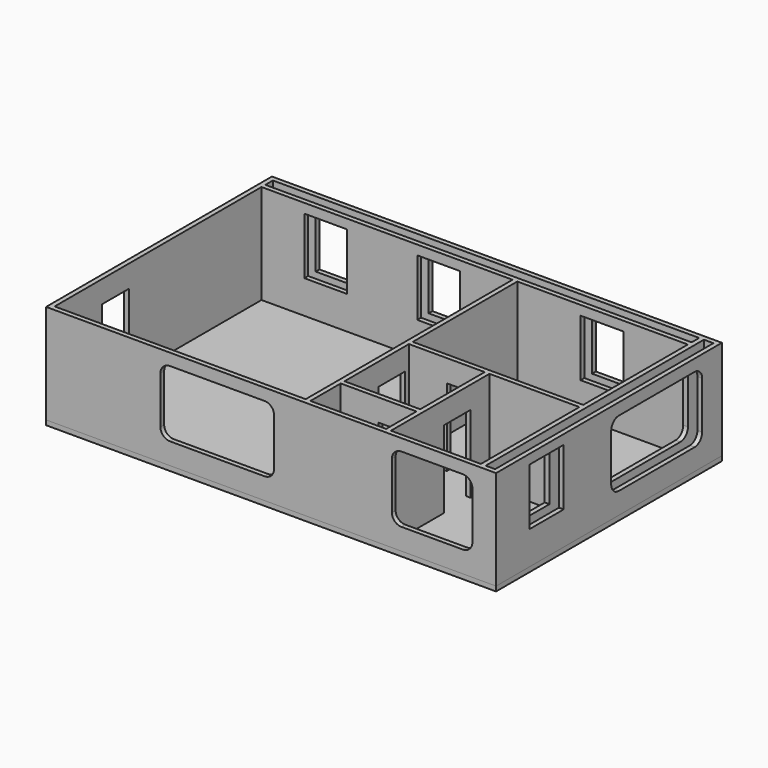
from build123d import *

# Parameters (mm, degrees)
F0_W      = 475
F0_H      = 298
F1_DEPTH  = 5
F2_W      = 475
F2_H      = 298
F2_W_2    = 80
F2_H_2    = 5
F3_DEPTH  = 105
F4_W      = 45
F4_H      = 60
F5_DEPTH  = 20
F7_DEPTH  = 5
F8_W      = 45
F8_H      = 60
F9_DEPTH  = 20
F10_W     = 35
F10_H     = 81.6
F11_DEPTH = 5
F12_W     = 35
F12_H     = 81.6
F13_DEPTH = 5
F14_W     = 35
F14_H     = 81.6
F15_DEPTH = 5
F16_W     = 35
F16_H     = 81.6
F17_DEPTH = 5
F18_W     = 35
F18_H     = 81.6
F19_DEPTH = 5


# Not quite as in the source:
# - a feature names something its author has since deleted; it is built from what else it names


with BuildPart() as f1:
    # F0 (on Top) → F1 (new body)
    with BuildSketch(Plane.XY):
        Rectangle(F0_W, F0_H)
    extrude(amount=-F1_DEPTH)


with BuildPart() as f3:
    # F2 (on face) → F3 (new body)
    with BuildSketch(Plane.XY):
        Rectangle(F2_W, F2_H)
        Polygon((232.5, 144), (232.5, -144), (222.5, -144), (217.5, -144), (122.5, -144), (117.5, -144), (37.5, -144), (32.5, -144), (-232.5, -144), (-232.5, 129), (-232.5, 134), (-232.5, 144), (217.5, 144), (222.5, 144), align=None, mode=Mode.SUBTRACT)
        Polygon((217.5, 129), (217.5, 134), (-232.5, 134), (-232.5, 129), (32.5, 129), (37.5, 129), align=None)
        Polygon((32.5, -144), (37.5, -144), (37.5, -104), (37.5, -99), (37.5, -14), (37.5, -9), (37.5, 129), (32.5, 129), align=None)
        Polygon((217.5, -144), (222.5, -144), (222.5, 144), (217.5, 144), (217.5, 134), (217.5, 129), (217.5, -9), (217.5, -14), align=None)
        Polygon((117.5, -144), (122.5, -144), (122.5, -14), (117.5, -14), (117.5, -99), (117.5, -104), align=None)
        Polygon((122.5, -14), (217.5, -14), (217.5, -9), (37.5, -9), (37.5, -14), (117.5, -14), align=None)
        with Locations((77.5, -101.5)):
            Rectangle(F2_W_2, F2_H_2)
    extrude(amount=F3_DEPTH)

    # F4 (on face) → F5 (cut, through all)
    with BuildSketch(Plane(origin=(0, 149, 0), x_dir=(-1, 0, 0), z_dir=(0, 1, 0))):
        with Locations((164.8025205731, 65)):
            Rectangle(F4_W, F4_H)
        with Locations((-126.8706479669, 65)):
            Rectangle(F4_W, F4_H)
        with Locations((45.589773953, 65)):
            Rectangle(F4_W, F4_H)
    extrude(amount=-F5_DEPTH, mode=Mode.SUBTRACT)

    # F6 (on face) → F7 (cut, through all)
    with BuildSketch(Plane.XZ.offset(149)):
        with BuildLine():
            ThreePointArc((3.1862647831, 82.5802037477), (0.257332595, 89.6512715596), (-6.8137352169, 92.5802037477))
            Line((-6.8137352169, 92.5802037477), (-106.8137352169, 92.5802037477))
            ThreePointArc((-106.8137352169, 92.5802037477), (-113.8848030287, 89.6512715596), (-116.8137352169, 82.5802037477))
            Line((-116.8137352169, 82.5802037477), (-116.8137352169, 32.5802037477))
            ThreePointArc((-116.8137352169, 32.5802037477), (-113.8848030287, 25.5091359359), (-106.8137352169, 22.5802037477))
            Line((-106.8137352169, 22.5802037477), (-6.8137352169, 22.5802037477))
            ThreePointArc((-6.8137352169, 22.5802037477), (0.257332595, 25.5091359359), (3.1862647831, 32.5802037477))
            Line((3.1862647831, 32.5802037477), (3.1862647831, 82.5802037477))
        make_face()
        with BuildLine():
            Line((202.5, 92.5802037477), (137.5, 92.5802037477))
            ThreePointArc((137.5, 92.5802037477), (130.4289321881, 89.6512715596), (127.5, 82.5802037477))
            Line((127.5, 82.5802037477), (127.5, 32.5802037477))
            ThreePointArc((127.5, 32.5802037477), (130.4289321881, 25.5091359359), (137.5, 22.5802037477))
            Line((137.5, 22.5802037477), (202.5, 22.5802037477))
            ThreePointArc((202.5, 22.5802037477), (209.5710678119, 25.5091359359), (212.5, 32.5802037477))
            Line((212.5, 32.5802037477), (212.5, 82.5802037477))
            ThreePointArc((212.5, 82.5802037477), (209.5710678119, 89.6512715596), (202.5, 92.5802037477))
        make_face()
    extrude(amount=-F7_DEPTH, mode=Mode.SUBTRACT)

    # F8 (on face) → F9 (cut, through all)
    with BuildSketch(Plane.YZ.offset(237.5)):
        with Locations((-82.2980084391, 65)):
            Rectangle(F8_W, F8_H)
        with BuildLine():
            Line((112.9197687081, 92.5802037477), (12.9197687081, 92.5802037477))
            ThreePointArc((12.9197687081, 92.5802037477), (5.8487008962, 89.6512715596), (2.9197687081, 82.5802037477))
            Line((2.9197687081, 82.5802037477), (2.9197687081, 32.5802037477))
            ThreePointArc((2.9197687081, 32.5802037477), (5.8487008962, 25.5091359359), (12.9197687081, 22.5802037477))
            Line((12.9197687081, 22.5802037477), (112.9197687081, 22.5802037477))
            ThreePointArc((112.9197687081, 22.5802037477), (119.9908365199, 25.5091359359), (122.9197687081, 32.5802037477))
            Line((122.9197687081, 32.5802037477), (122.9197687081, 82.5802037477))
            ThreePointArc((122.9197687081, 82.5802037477), (119.9908365199, 89.6512715596), (112.9197687081, 92.5802037477))
        make_face()
    extrude(amount=-F9_DEPTH, mode=Mode.SUBTRACT)

    # F10 (on face) → F11 (cut, through all)
    with BuildSketch(Plane.YZ.offset(37.5)):
        with Locations((-36.5, 40.8)):
            Rectangle(F10_W, F10_H)
    extrude(amount=-F11_DEPTH, mode=Mode.SUBTRACT)

    # F12 (on face) → F13 (cut, through all)
    with BuildSketch(Plane(origin=(117.5, 0, 0), x_dir=(0, -1, 0), z_dir=(-1, 0, 0))):
        with Locations((56.5, 40.8)):
            Rectangle(F12_W, F12_H)
    extrude(amount=-F13_DEPTH, mode=Mode.SUBTRACT)

    # F14 (on face) → F15 (cut, through all)
    with BuildSketch(Plane.XZ.offset(104)):
        with Locations((95, 40.8)):
            Rectangle(F14_W, F14_H)
    extrude(amount=-F15_DEPTH, mode=Mode.SUBTRACT)

    # F16 (on face) → F17 (cut, through all)
    with BuildSketch(Plane.XZ.offset(14)):
        with Locations((95, 40.8)):
            Rectangle(F16_W, F16_H)
    extrude(amount=-F17_DEPTH, mode=Mode.SUBTRACT)

    # F18 (on face) → F19 (cut, through all)
    with BuildSketch(Plane(origin=(-237.5, 0, 0), x_dir=(0, -1, 0), z_dir=(-1, 0, 0))):
        with Locations((63.6425632238, 40.8)):
            Rectangle(F18_W, F18_H)
    extrude(amount=-F19_DEPTH, mode=Mode.SUBTRACT)


solid = Compound([f1.part, f3.part])
